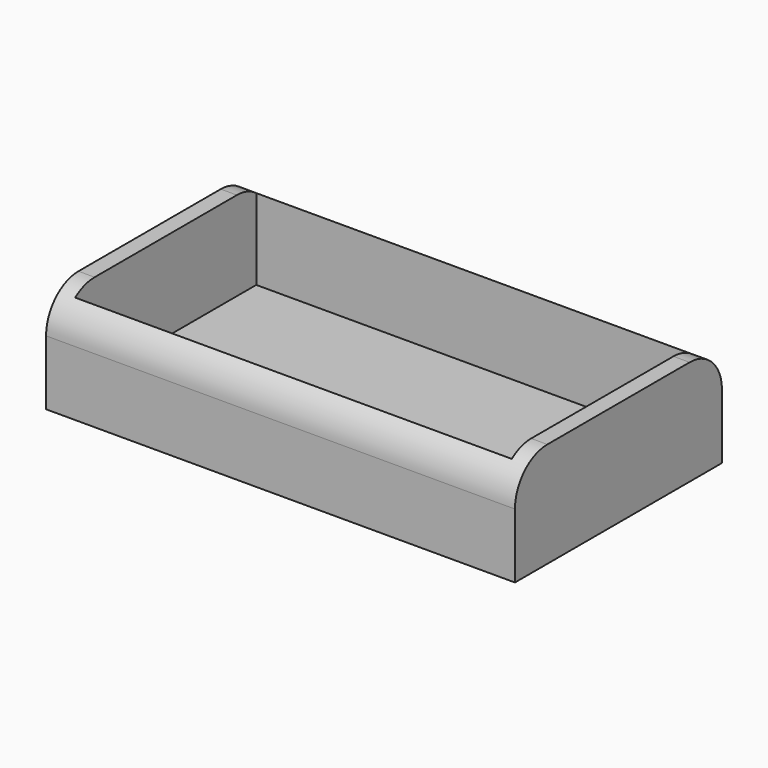
from build123d import *

# Parameters (mm, degrees)
F0_W        = 58
F0_H        = 32
F1_DEPTH    = 13
F2_T        = -2
F3_T1_DEPTH = 83


# Not quite as in the source:
# - a fillet or chamfer that OpenCascade refuses, or shapes differently, is made with other operations: its cross-section is extruded or revolved along the edge and cut away or added


with BuildPart() as f1:
    # F0 (on Top) → F1 (new body)
    with BuildSketch(Plane.XY):
        with Locations((29, 16)):
            Rectangle(F0_W, F0_H)
    extrude(amount=F1_DEPTH)

    # F2
    f2_openings = [f1.faces().sort_by_distance(p)[0] for p in [
        (29, 16, 13),
    ]]
    offset(amount=F2_T, openings=f2_openings)

    # F3: fillet of radius 5 on 2 edges, made by hand

    # F3_s2 → F3_t1 (cut)
    with BuildSketch(Plane.YZ.offset(-12.5)):
        with BuildLine():
            ThreePointArc((0, 8), (1.4644660941, 11.5355339059), (5, 13))
            Line((5, 13), (0, 13))
            Line((0, 13), (0, 8))
        make_face()
        with BuildLine():
            ThreePointArc((32, 8), (30.5355339059, 11.5355339059), (27, 13))
            Line((27, 13), (32, 13))
            Line((32, 13), (32, 8))
        make_face()
    extrude(amount=F3_T1_DEPTH, mode=Mode.SUBTRACT)


solid = f1.part
